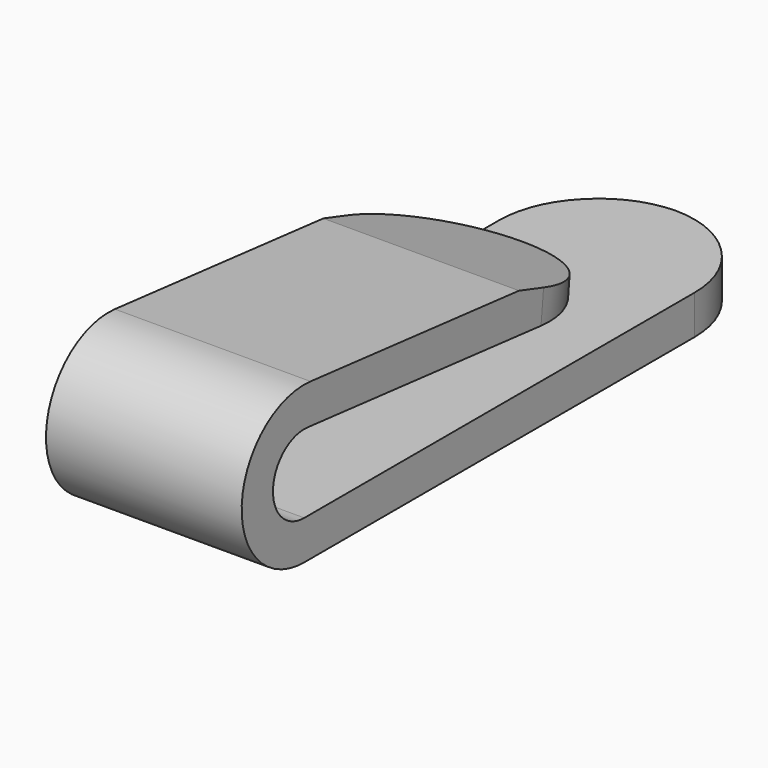
from build123d import *

# Parameters (mm, degrees)
F1_DEPTH    = 5
F2_SIZE     = 3
F3_T1_DEPTH = 12.3553390593
F3_T3_DEPTH = 13.1207993933


# Not quite as in the source:
# - a fillet or chamfer that OpenCascade refuses, or shapes differently, is made with other operations: its cross-section is extruded or revolved along the edge and cut away or added


with BuildPart() as f1:
    # F0 (on Right) → F1 (new body, symmetric)
    with BuildSketch(Plane.YZ):
        with BuildLine():
            Line((11.971969828, -2), (11.971969828, 0))
            Line((11.971969828, 0), (-18.028030172, 0))
            ThreePointArc((-18.028030172, 0), (-20.0255447559, 2.0996769133), (-17.828924084, 3.990064513))
            Line((-17.828924084, 3.990064513), (2.0717210456, 1.9990036332))
            Line((2.0717210456, 1.9990036332), (2.1335235149, 2.6167190544))
            Line((2.1335235149, 2.6167190544), (-4.3118495071, 4.6476653855))
            Line((-4.3118495071, 4.6476653855), (-17.629817996, 5.9801290259))
            ThreePointArc((-17.629817996, 5.9801290259), (-22.0230593398, 2.1993538266), (-18.028030172, -2))
            Line((-18.028030172, -2), (11.971969828, -2))
        make_face()
    extrude(amount=F1_DEPTH, both=True)

    # F2
    f2_edges = [f1.edges().sort_by_distance(p)[0] for p in [
        (5, 11.97197, -1),
        (-5, 11.97197, -1),
    ]]
    chamfer(f2_edges, length=F2_SIZE)

    # F3: fillet of radius 5 on 6 edges, made by hand

    # F3_s2 → F3_t1 (cut)
    with BuildSketch(Plane.XY.offset(-7.1776695297)):
        with BuildLine():
            ThreePointArc((-3.5355339059, 10.4364359221), (-4.6193976626, 8.814319178), (-5, 6.9009020161))
            Line((-5, 6.9009020161), (-5, 8.971969828))
            Line((-5, 8.971969828), (-3.5355339059, 10.4364359221))
        make_face()
        with BuildLine():
            ThreePointArc((0.0710678119, 11.971969828), (-1.84234935, 11.5913674906), (-3.4644660941, 10.5075037339))
            Line((-3.4644660941, 10.5075037339), (-2, 11.971969828))
            Line((-2, 11.971969828), (0.0710678119, 11.971969828))
        make_face()
        with BuildLine():
            ThreePointArc((-0.0710678119, 11.971969828), (1.84234935, 11.5913674906), (3.4644660941, 10.5075037339))
            Line((3.4644660941, 10.5075037339), (2, 11.971969828))
            Line((2, 11.971969828), (-0.0710678119, 11.971969828))
        make_face()
        with BuildLine():
            ThreePointArc((3.5355339059, 10.4364359221), (4.6193976626, 8.814319178), (5, 6.9009020161))
            Line((5, 6.9009020161), (5, 8.971969828))
            Line((5, 8.971969828), (3.5355339059, 10.4364359221))
        make_face()
    extrude(amount=F3_T1_DEPTH, mode=Mode.SUBTRACT)

    # F3_s4 → F3_t3 (cut)
    with BuildSketch(Plane(origin=(0, 0.2185507121, 2.1844134494), x_dir=(1, 0, 0), z_dir=(0, 0.099553044, 0.9950322565))):
        with BuildLine():
            ThreePointArc((-5, -3.1375776299), (-3.5355339059, 0.3979562761), (0, 1.8624223701))
            Line((0, 1.8624223701), (-5, 1.8624223701))
            Line((-5, 1.8624223701), (-5, -3.1375776299))
        make_face()
        with BuildLine():
            ThreePointArc((5, -3.1375776299), (3.5355339059, 0.3979562761), (0, 1.8624223701))
            Line((0, 1.8624223701), (5, 1.8624223701))
            Line((5, 1.8624223701), (5, -3.1375776299))
        make_face()
    extrude(amount=F3_T3_DEPTH, mode=Mode.SUBTRACT)


solid = f1.part
